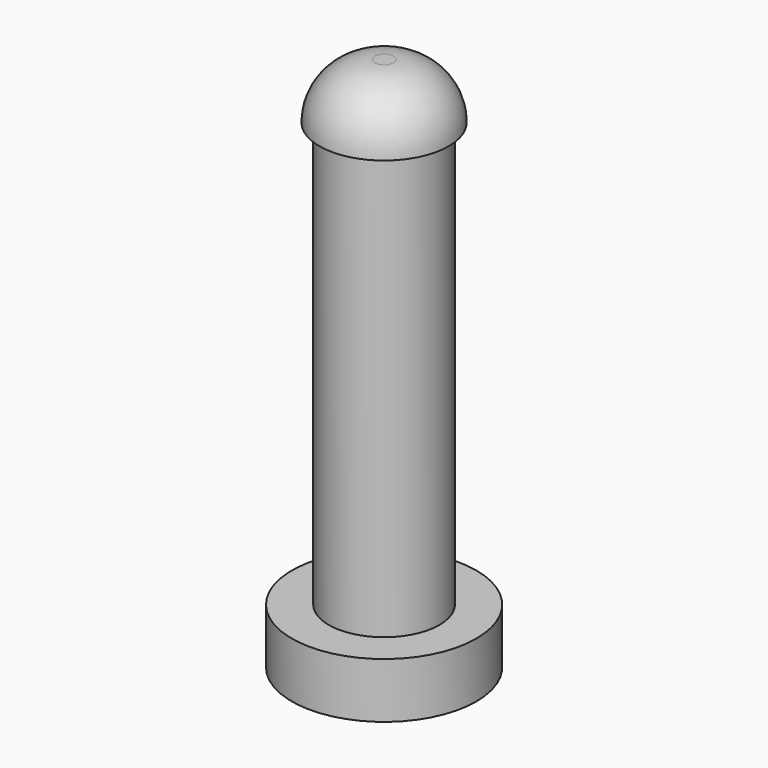
from build123d import *

# Parameters (mm, degrees)
F0_R     = 1.5
F1_DEPTH = 13
F0_R_2   = 2.5
F2_DEPTH = 1.5
F3_R     = 1.75
F4_DEPTH = 1.5
F5_R     = 1.49999


# Not quite as in the source:
# - a fillet or chamfer is up to 0.001 mm smaller than in the source, because OpenCascade refuses the exact size


with BuildPart() as f1:
    # F0 (on Top) → F1 (new body)
    with BuildSketch(Plane.XY):
        Circle(F0_R)
    extrude(amount=F1_DEPTH)

    # F0 (on Top) → F2 (join)
    with BuildSketch(Plane.XY):
        Circle(F0_R_2)
        Circle(F0_R, mode=Mode.SUBTRACT)
    extrude(amount=F2_DEPTH)

    # F3 (on face) → F4 (join)
    with BuildSketch(Plane.XY.offset(13)):
        Circle(F3_R)
    extrude(amount=F4_DEPTH)

    # F5 (radius 1.5 in the source; OpenCascade refuses exactly that, so slightly less here)
    f5_edges = [f1.edges().sort_by_distance(p)[0] for p in [
        (-1.75, 0, 14.5),
    ]]
    fillet(f5_edges, radius=F5_R)


solid = f1.part
